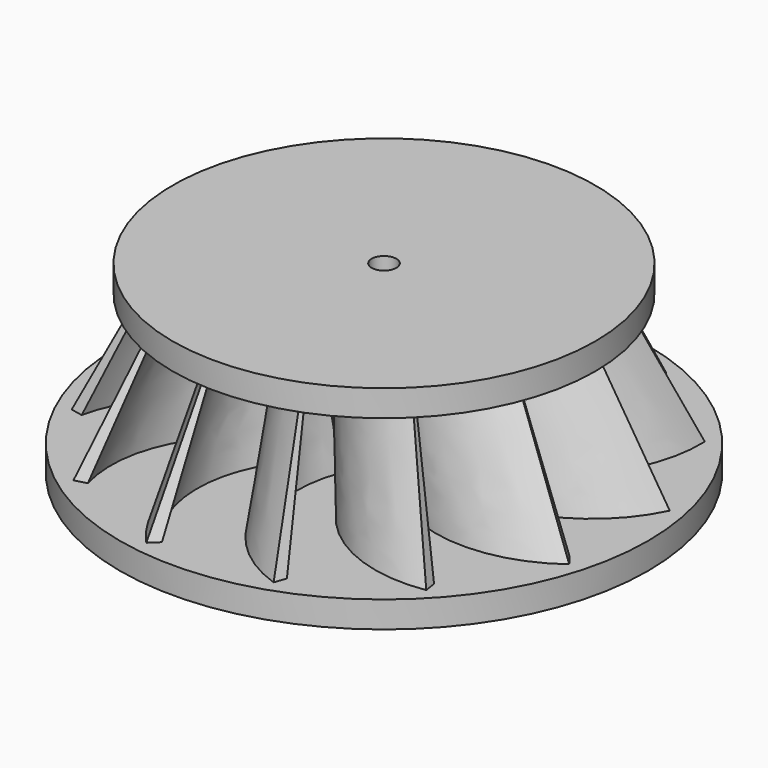
from build123d import *

# Parameters (mm, degrees)
F0_R      = 50.8
F0_R_2    = 3.175
F1_DEPTH  = 5.08
F6_COUNT  = 13
F7_R      = 40.64
F7_R_2    = 2.374766436
F9_DEPTH  = 5.08
F8_R      = 7.3667190134
F8_R_2    = 3.2527268044
F10_DEPTH = 16.764


# Not quite as in the source:
# - a fillet or chamfer that OpenCascade refuses, or shapes differently, is made with other operations: its cross-section is extruded or revolved along the edge and cut away or added


with BuildPart() as f1:
    # F0 (on Top) → F1 (new body)
    with BuildSketch(Plane.XY):
        Circle(F0_R)
        Circle(F0_R_2, mode=Mode.SUBTRACT)
    extrude(amount=F1_DEPTH)

    # F4 (on offset) → F5 section 0
    with BuildSketch(Plane.XY.offset(30.48)):
        with BuildLine():
            ThreePointArc((-31.2581645276, -15.0454975722), (-23.8275721708, -2.3651081034), (-10.6147182313, 4.0712317435))
            Line((-10.6147182313, 4.0712317435), (-10.4037430393, 4.9518312593))
            ThreePointArc((-10.4037430393, 4.9518312593), (-24.2782382092, -1.6407206053), (-32.0789483615, -14.873720168))
            Line((-32.0789483615, -14.873720168), (-31.2581645276, -15.0454975722))
        make_face()
    # F2 (on face) → F5 section 1
    with BuildSketch(Plane.XY.offset(5.08)):
        with BuildLine():
            Line((-11.3569097297, -2.2971912867), (-10.8065456152, 0))
            ThreePointArc((-10.8065456152, 0), (-31.5323680256, -3.4460367679), (-43.5032732785, -20.7125451416))
            Line((-43.5032732785, -20.7125451416), (-41.1911659165, -21.1964335717))
            ThreePointArc((-41.1911659165, -21.1964335717), (-30.2682669102, -5.4415409238), (-11.3569097297, -2.2971912867))
        make_face()
    loft()


with BuildPart() as f6_1:
    # F6: instance of F1
    add(f1.part.rotate(Axis((0, 0, 5.08), (0, 0, 1)), 1 * 360 / F6_COUNT))


with BuildPart() as f6_2:
    # F6: instance of F1
    add(f1.part.rotate(Axis((0, 0, 5.08), (0, 0, 1)), 2 * 360 / F6_COUNT))


with BuildPart() as f6_3:
    # F6: instance of F1
    add(f1.part.rotate(Axis((0, 0, 5.08), (0, 0, 1)), 3 * 360 / F6_COUNT))


with BuildPart() as f6_4:
    # F6: instance of F1
    add(f1.part.rotate(Axis((0, 0, 5.08), (0, 0, 1)), 4 * 360 / F6_COUNT))


with BuildPart() as f6_5:
    # F6: instance of F1
    add(f1.part.rotate(Axis((0, 0, 5.08), (0, 0, 1)), 5 * 360 / F6_COUNT))


with BuildPart() as f6_6:
    # F6: instance of F1
    add(f1.part.rotate(Axis((0, 0, 5.08), (0, 0, 1)), 6 * 360 / F6_COUNT))


with BuildPart() as f6_7:
    # F6: instance of F1
    add(f1.part.rotate(Axis((0, 0, 5.08), (0, 0, 1)), 7 * 360 / F6_COUNT))


with BuildPart() as f6_8:
    # F6: instance of F1
    add(f1.part.rotate(Axis((0, 0, 5.08), (0, 0, 1)), 8 * 360 / F6_COUNT))


with BuildPart() as f6_9:
    # F6: instance of F1
    add(f1.part.rotate(Axis((0, 0, 5.08), (0, 0, 1)), 9 * 360 / F6_COUNT))


with BuildPart() as f6_10:
    # F6: instance of F1
    add(f1.part.rotate(Axis((0, 0, 5.08), (0, 0, 1)), 10 * 360 / F6_COUNT))


with BuildPart() as f6_11:
    # F6: instance of F1
    add(f1.part.rotate(Axis((0, 0, 5.08), (0, 0, 1)), 11 * 360 / F6_COUNT))


with BuildPart() as f6_12:
    # F6: instance of F1
    add(f1.part.rotate(Axis((0, 0, 5.08), (0, 0, 1)), 12 * 360 / F6_COUNT))


with BuildPart() as f1_1:
    add(f1.part)

    add(f6_1.part)  # F9 merges F6_1

    add(f6_2.part)  # F9 merges F6_2

    add(f6_3.part)  # F9 merges F6_3

    add(f6_4.part)  # F9 merges F6_4

    add(f6_5.part)  # F9 merges F6_5

    add(f6_6.part)  # F9 merges F6_6

    add(f6_7.part)  # F9 merges F6_7

    add(f6_8.part)  # F9 merges F6_8

    add(f6_9.part)  # F9 merges F6_9

    add(f6_10.part)  # F9 merges F6_10

    add(f6_11.part)  # F9 merges F6_11

    add(f6_12.part)  # F9 merges F6_12
    # F7 (on offset) → F9 (join)
    with BuildSketch(Plane.XY.offset(30.48)):
        Circle(F7_R)
        Circle(F7_R_2, mode=Mode.SUBTRACT)
    extrude(amount=F9_DEPTH)

    # F8 (on face) → F10 (join)
    with BuildSketch(Plane.XY.offset(5.08)):
        Circle(F8_R)
        Circle(F8_R_2, mode=Mode.SUBTRACT)
    extrude(amount=F10_DEPTH)

    # F11: fillet of radius 5.08 on 1 edges, made by hand

    # F11_s1 → F11_t2 (revolve, cut)
    with BuildSketch(Plane.XZ):
        with BuildLine():
            ThreePointArc((7.3667190134, 16.856693217), (6.2055019608, 20.0892680747), (3.2527268044, 21.844))
            Line((3.2527268044, 21.844), (7.3667190134, 21.844))
            Line((7.3667190134, 21.844), (7.3667190134, 16.856693217))
        make_face()
    revolve(axis=Axis((0, 0, 21.844), (0, 0, 1)), mode=Mode.SUBTRACT)


solid = f1_1.part
